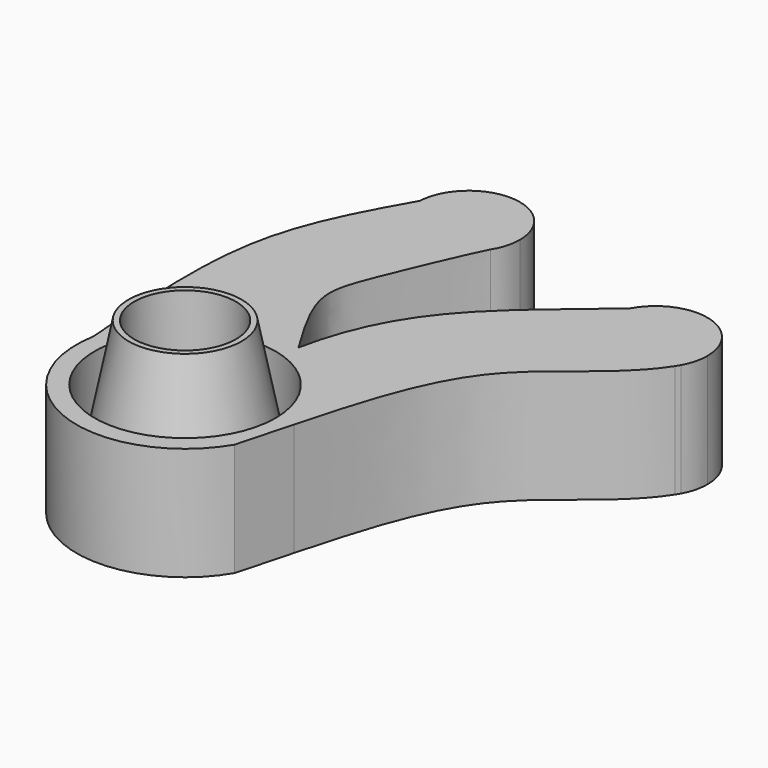
from build123d import *

# Parameters (mm, degrees)
F0_R     = 16
F2_R     = 10
F4_T     = -3
F5_DEPTH = 20
F6_D     = 18
F6_DEPTH = 10
F6_TIP   = 5.4077455712
F7_D     = 32
F7_DEPTH = 0.5
F7_TIP   = 9.6137699044


# Not quite as in the source:
# - a feature names something its author has since deleted; it is built from what else it names


with BuildPart() as f3:
    # F0 (on Top) → F3 section 0
    with BuildSketch(Plane.XY):
        Circle(F0_R)
    # F2 (on offset) → F3 section 1
    with BuildSketch(Plane.XY.offset(30)):
        Circle(F2_R)
    loft()

    # F4 (hollow: no face is removed)
    offset(amount=F4_T, mode=Mode.SUBTRACT)

    # F6
    with Locations(Plane.XY.offset(30)):
        with Locations((0, 0)):
            Hole(F6_D / 2, depth=F6_DEPTH)
            with Locations((0, 0, -(F6_DEPTH + F6_TIP / 2))):  # 118° drill point
                Cone(0, F6_D / 2, F6_TIP, mode=Mode.SUBTRACT)

    # F7
    with Locations(Plane(origin=(0, 0, 0), x_dir=(1, 0, 0), z_dir=(0, 0, -1))):
        with Locations((0, 0)):
            Hole(F7_D / 2, depth=F7_DEPTH)
            with Locations((0, 0, -(F7_DEPTH + F7_TIP / 2))):  # 118° drill point
                Cone(0, F7_D / 2, F7_TIP, mode=Mode.SUBTRACT)


with BuildPart() as f5:
    # F0 (on Top) → F5 (new body)
    with BuildSketch(Plane.XY):
        with BuildLine():
            ThreePointArc((19.1937116741, 0.1042258071), (15.2991489183, 11.5907494677), (5.2955546416, 18.4490252286))
            ThreePointArc((5.2955546416, 18.4490252286), (-10.1587733981, 16.2852311588), (-18.8981625306, 3.3569158189))
            ThreePointArc((-18.8981625306, 3.3569158189), (-6.6406726309, -18.0086339809), (16.5533281406, -9.7157994173))
            add(Edge.make_bspline(
                [(16.5533281406, -9.7157994173), (17.4909471556, -6.282790694), (18.3547028822, -3.0072993549), (19.1937116741, 0.1042258071)],
                knots=[0, 0, 0, 0, 0.1115447748, 0.1115447748, 0.1115447748, 0.1115447748], degree=3))
        make_face()
        Circle(F0_R, mode=Mode.SUBTRACT)
        with BuildLine():
            add(Edge.make_bspline(
                [(5.2955546416, 18.4490252286), (7.1746227331, 27.6735369116), (14.3114232279, 40.9606919462), (27.690502152, 50.9134689797), (33.7236113846, 56.2075078487)],
                knots=[0, 0, 0, 0, 0.5007148854, 1, 1, 1, 1], degree=3))
            ThreePointArc((5.2955546416, 18.4490252286), (15.2991489183, 11.5907494677), (19.1937116741, 0.1042258071))
            add(Edge.make_bspline(
                [(19.1937116741, 0.1042258071), (22.5582500765, 12.5818613195), (28.3536912987, 31.8067560439), (44.7186086588, 39.3813644075), (49.3468357907, 46.577233643)],
                knots=[0.1115447748, 0.1115447748, 0.1115447748, 0.1115447748, 0.5588543644, 0.9853987705, 0.9853987705, 0.9853987705, 0.9853987705], degree=3))
            ThreePointArc((49.3468357907, 46.577233643), (36.9461417786, 43.9474887633), (33.7236113846, 56.2075078487))
        make_face()
        with BuildLine():
            ThreePointArc((-18.8981625306, 3.3569158189), (-10.1587733981, 16.2852311588), (5.2955546416, 18.4490252286))
            add(Edge.make_bspline(
                [(5.2955546416, 18.4490252286), (-2.5623629335, 31.2608480453), (-2.628851385, 35.2579723672), (7.0271153581, 56.848888653), (7.6760536531, 57.9190816164)],
                knots=[0, 0, 0, 0, 0.5180671246, 0.9957919408, 0.9957919408, 0.9957919408, 0.9957919408], degree=3))
            ThreePointArc((7.6760536531, 57.9190816164), (-2.7140834876, 54.0759145506), (-9.0335700658, 63.1747591085))
            add(Edge.make_bspline(
                [(-18.8981625306, 3.3569158189), (-20.0090761688, 16.85842438), (-21.9506635835, 40.1142274591), (-13.0991634095, 56.0064077769), (-9.0335700658, 63.1747591085)],
                knots=[0, 0, 0, 0, 0.5477086796, 1, 1, 1, 1], degree=3))
        make_face()
        with BuildLine():
            ThreePointArc((-9.0335700658, 63.1747591085), (-2.7140834876, 54.0759145506), (7.6760536531, 57.9190816164))
            ThreePointArc((7.6760536531, 57.9190816164), (7.6841733008, 57.9321294513), (7.6922707696, 57.9451910618))
            ThreePointArc((7.6922707696, 57.9451910618), (8.7008251114, 60.2307070152), (9.0457796257, 62.704928391))
            ThreePointArc((9.0457796257, 62.704928391), (0.2349946683, 71.7476551115), (-9.0335700658, 63.1747591085))
        make_face()
        with BuildLine():
            ThreePointArc((50.9538851021, 51.7681334168), (44.0590251845, 60.6646267952), (33.7236113846, 56.2075078487))
            ThreePointArc((33.7236113846, 56.2075078487), (36.9461417786, 43.9474887633), (49.3468357907, 46.577233643))
            add(Edge.make_bspline(
                [(49.3468357907, 46.577233643), (49.5052666724, 46.8235586126), (49.6597605763, 47.0739831673), (49.8100817204, 47.3287589848)],
                knots=[0.9853987705, 0.9853987705, 0.9853987705, 0.9853987705, 1, 1, 1, 1], degree=3))
            ThreePointArc((49.8100817204, 47.3287589848), (50.6633399309, 49.4759547848), (50.9538851021, 51.7681334168))
        make_face()
    extrude(amount=F5_DEPTH)


solid = Compound([f3.part, f5.part])
